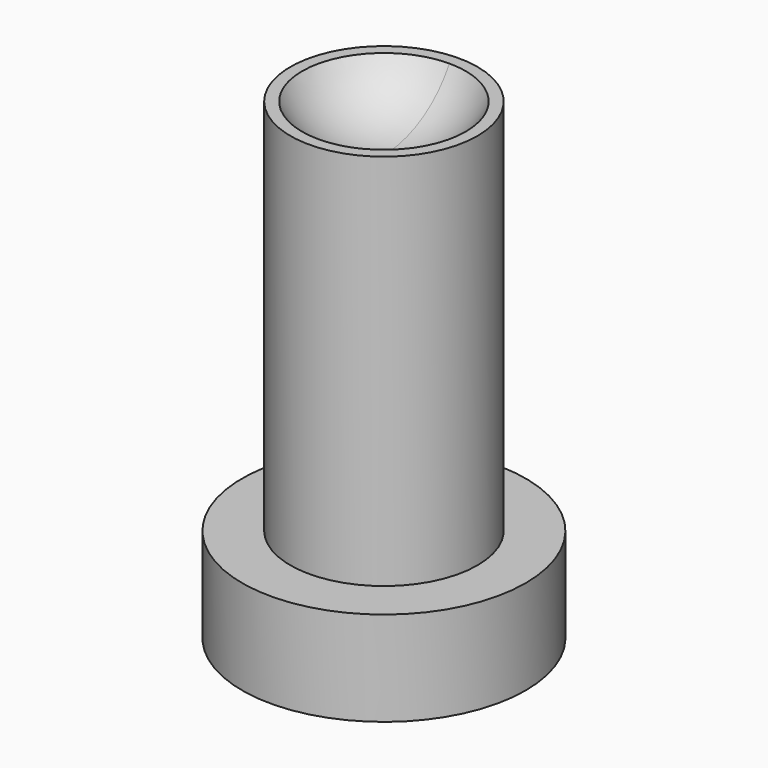
from build123d import *
from build123d import SkipClean  # not in build123d's __all__

# Parameters (mm, degrees)
F0_R     = 19.05
F1_DEPTH = 12.7
F2_R     = 12.573
F3_DEPTH = 50.8


with BuildPart() as f1:
    # F0 (on Top) → F1 (new body)
    with BuildSketch(Plane.XY):
        Circle(F0_R)
    extrude(amount=F1_DEPTH)

    # F2 (on face) → F3 (join)
    with BuildSketch(Plane.XY.offset(12.7)):
        Circle(F2_R)
    extrude(amount=F3_DEPTH)

    # F4 (on Right) → F5 (revolve, cut)
    with BuildSketch(Plane.YZ):
        with BuildLine():
            Line((12.7, 69.85), (-12.7, 69.85))
            ThreePointArc((-12.7, 69.85), (0, 57.15), (12.7, 69.85))
        make_face()
    with SkipClean():  # cleaning this boolean's faces spoils the solid; the shape is the same uncleaned
        revolve(axis=Axis((0, 0, 69.85), (0, -1, 0)), mode=Mode.SUBTRACT)


solid = f1.part
